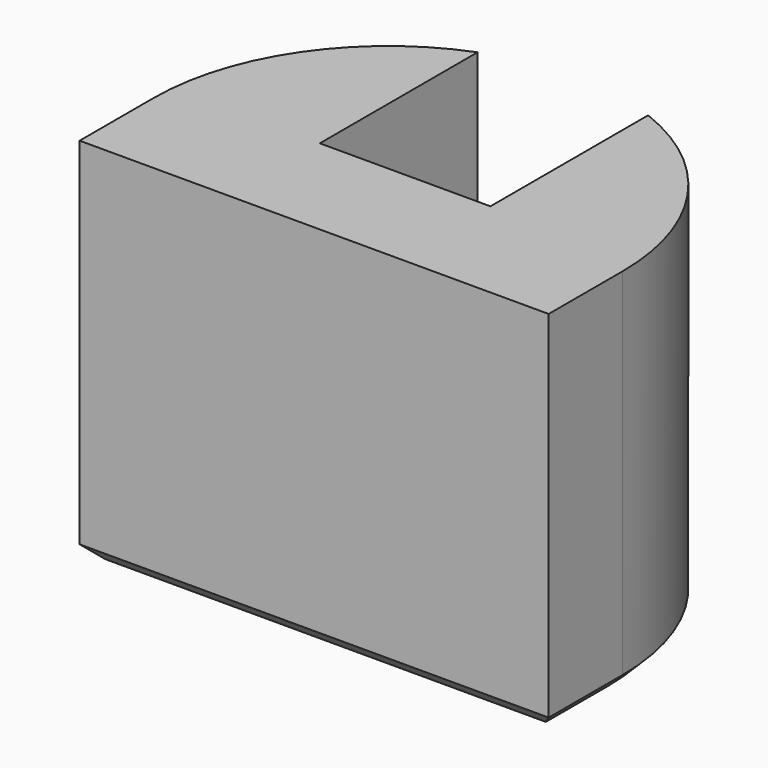
from build123d import *

# Parameters (mm, degrees)
F4_DEPTH  = 1
F6_DEPTH  = 12
F7_SIZE   = 0.5
F8_W      = 6
F8_H      = 3
F9_DEPTH  = 12
F10_DEPTH = 5
F11_W     = 6
F11_H     = 1.5
F12_DEPTH = 1
F13_SIZE  = 0.99999


# Not quite as in the source:
# - a fillet or chamfer is up to 0.001 mm smaller than in the source, because OpenCascade refuses the exact size


with BuildPart() as f4:
    # F3 (on Top) → F4 (new body)
    with BuildSketch(Plane.XY):
        with BuildLine():
            Line((-8.25, 0), (0, 0))
            Line((0, 0), (8.25, 0))
            Line((8.25, 0), (8.25, 3.25))
            ThreePointArc((8.25, 3.25), (0, 11.5), (-8.25, 3.25))
            Line((-8.25, 3.25), (-8.25, 0))
        make_face()
    extrude(amount=F4_DEPTH)

    # F5 (on face) → F6 (join)
    with BuildSketch(Plane.XY.offset(1)):
        with BuildLine():
            Line((-3, 0), (-3, 10.9352130745))
            ThreePointArc((-3, 10.9352130745), (-6.8122132967, 7.9036276172), (-8.25, 3.25))
            Line((-8.25, 3.25), (-8.25, 0))
            Line((-8.25, 0), (-3, 0))
        make_face()
        with BuildLine():
            ThreePointArc((8.25, 3.25), (6.8122132967, 7.9036276172), (3, 10.9352130745))
            Line((3, 10.9352130745), (3, 0))
            Line((3, 0), (8.25, 0))
            Line((8.25, 0), (8.25, 3.25))
        make_face()
    extrude(amount=F6_DEPTH)

    # F7
    f7_edges = [f4.edges().sort_by_distance(p)[0] for p in [
        (8.25, 1.625, 0),
        (0, 0, 0),
    ]]
    chamfer(f7_edges, length=F7_SIZE)

    # F8 (on face) → F9 (join)
    with BuildSketch(Plane.XY.offset(1)):
        with Locations((0, 1.5)):
            Rectangle(F8_W, F8_H)
    extrude(amount=F9_DEPTH)

    # F10 (add): a face of the model
    f10_faces = [f4.faces().sort_by_distance(p)[0] for p in [
        (0, 7.1588841066, 1),
    ]]
    extrude(f10_faces, amount=F10_DEPTH)

    # F11 (on face) → F12 (join)
    with BuildSketch(Plane(origin=(0, 3, 0), x_dir=(-1, 0, 0), z_dir=(0, 1, 0))):
        with Locations((0, 12.25)):
            Rectangle(F11_W, F11_H)
    extrude(amount=F12_DEPTH)

    # F13 (size 1 in the source; OpenCascade refuses exactly that, so slightly less here)
    f13_edges = [f4.edges().sort_by_distance(p)[0] for p in [
        (0, 4, 11.5),
    ]]
    chamfer(f13_edges, length=F13_SIZE)


solid = f4.part
